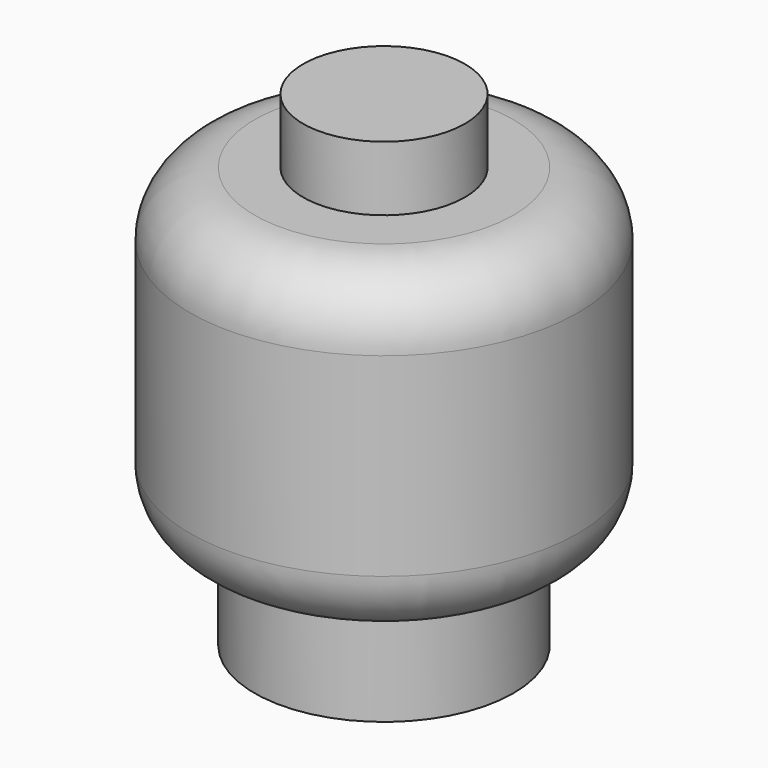
from build123d import *

# Parameters (mm, degrees)
F0_R     = 4
F1_DEPTH = 3
F2_R     = 6
F3_DEPTH = 10
F4_DEPTH = 8
F5_R     = 2.5
F6_DEPTH = 2
F7_R     = 1.99999
F8_R     = 2.5
F9_DEPTH = 8


# Not quite as in the source:
# - a fillet or chamfer is up to 0.001 mm smaller than in the source, because OpenCascade refuses the exact size


with BuildPart() as f1:
    # F0 (on Top) → F1 (new body)
    with BuildSketch(Plane.XY):
        Circle(F0_R)
    extrude(amount=F1_DEPTH)

    # F2 (on face) → F3 (join)
    with BuildSketch(Plane.XY.offset(3)):
        Circle(F2_R)
    extrude(amount=F3_DEPTH)

    # F2 (on face) → F4 (join)
    with BuildSketch(Plane.XY.offset(3)):
        Circle(F2_R)
    extrude(amount=F4_DEPTH)

    # F5 (on face) → F6 (join)
    with BuildSketch(Plane.XY.offset(13)):
        Circle(F5_R)
    extrude(amount=F6_DEPTH)

    # F7 (radius 2 in the source; OpenCascade refuses exactly that, so slightly less here)
    f7_edges = [f1.edges().sort_by_distance(p)[0] for p in [
        (-6, 0, 13),
        (-6, 0, 3),
    ]]
    fillet(f7_edges, radius=F7_R)

    # F8 (on face) → F9 (cut)
    with BuildSketch(Plane(origin=(0, 0, 0), x_dir=(1, 0, 0), z_dir=(0, 0, -1))):
        Circle(F8_R)
    extrude(amount=-F9_DEPTH, mode=Mode.SUBTRACT)


solid = f1.part
